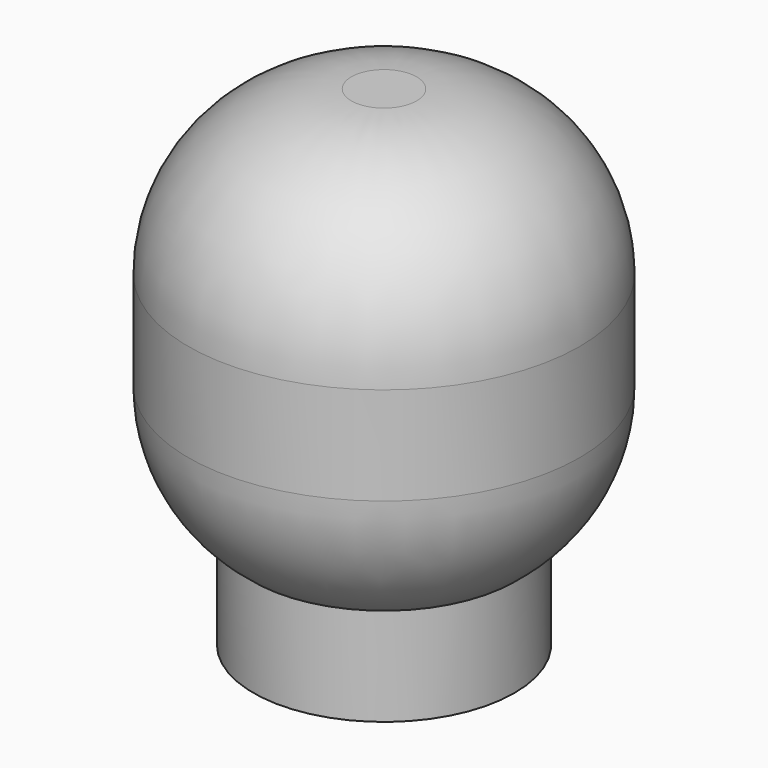
from build123d import *

# Parameters (mm, degrees)
F0_R     = 4
F1_DEPTH = 3
F2_R     = 6
F3_DEPTH = 12
F4_R     = 5
F6_R     = 2.5
F7_DEPTH = 8
F9_DEPTH = 8


# Not quite as in the source:
# - a fillet or chamfer that OpenCascade refuses, or shapes differently, is made with other operations: its cross-section is extruded or revolved along the edge and cut away or added


with BuildPart() as f1:
    # F0 (on Top) → F1 (new body)
    with BuildSketch(Plane.XY):
        Circle(F0_R)
    extrude(amount=F1_DEPTH)

    # F2 (on face) → F3 (join)
    with BuildSketch(Plane.XY.offset(3)):
        Circle(F2_R)
    extrude(amount=F3_DEPTH)

    # F4
    f4_edges = [f1.edges().sort_by_distance(p)[0] for p in [
        (-6, 0, 15),
    ]]
    fillet(f4_edges, radius=F4_R)

    # F5: fillet of radius 5 on 1 edges, made by hand

    # F5_s1 → F5_t2 (revolve, cut)
    with BuildSketch(Plane.XZ):
        with BuildLine():
            ThreePointArc((6, 7), (5.472135955, 4.7639320225), (4, 3))
            Line((4, 3), (6, 3))
            Line((6, 3), (6, 7))
        make_face()
    revolve(axis=Axis((0, 0, 3), (0, 0, 1)), mode=Mode.SUBTRACT)

    # F6 (on face) → F7 (cut)
    with BuildSketch(Plane(origin=(0, 0, 0), x_dir=(1, 0, 0), z_dir=(0, 0, -1))):
        Circle(F6_R)
    extrude(amount=-F7_DEPTH, mode=Mode.SUBTRACT)

    # F8 (on Front) → F9 (cut)
    with BuildSketch(Plane.XZ):
        with BuildLine():
            Line((-1.3463870705, 8.7240217328), (-1.3463870705, 8.3487899899))
            ThreePointArc((-1.3463870705, 8.3487899899), (-1.3369403935, 8.4423866045), (-1.3337867757, 8.5364058614))
            ThreePointArc((-1.3337867757, 8.5364058614), (-1.3369403935, 8.6304251183), (-1.3463870705, 8.7240217328))
        make_face()
        with BuildLine():
            ThreePointArc((-1.3337867757, 8.5364058614), (-1.3369403935, 8.4423866045), (-1.3463870705, 8.3487899899))
            Line((-1.3463870705, 8.3487899899), (1.4683810595, 8.3487899899))
            Line((1.4683810595, 8.3487899899), (1.4683810595, 8.5058610392))
            ThreePointArc((1.4683810595, 8.5058610392), (1.4637016301, 8.6179580539), (1.4683810595, 8.7300550686))
            Line((1.4683810595, 8.7300550686), (-1.3463870705, 8.7300550686))
            Line((-1.3463870705, 8.7300550686), (-1.3463870705, 8.7240217328))
            ThreePointArc((-1.3463870705, 8.7240217328), (-1.3369403935, 8.6304251183), (-1.3337867757, 8.5364058614))
        make_face()
        with BuildLine():
            ThreePointArc((-1.3463870705, 8.7240217328), (-4.1399498979, 8.5364058614), (-1.3463870705, 8.3487899899))
            Line((-1.3463870705, 8.3487899899), (-1.3463870705, 8.7240217328))
        make_face()
        with BuildLine():
            Line((1.4683810595, 8.7300550686), (1.4683810595, 8.5058610392))
            ThreePointArc((1.4683810595, 8.5058610392), (2.864796007, 7.2741313647), (4.1536957416, 8.6179580539))
            ThreePointArc((4.1536957416, 8.6179580539), (2.864796007, 9.9617847432), (1.4683810595, 8.7300550686))
        make_face()
        with BuildLine():
            ThreePointArc((1.4683810595, 8.7300550686), (1.4637016301, 8.6179580539), (1.4683810595, 8.5058610392))
            Line((1.4683810595, 8.5058610392), (1.4683810595, 8.7300550686))
        make_face()
    extrude(amount=-F9_DEPTH, mode=Mode.SUBTRACT)


solid = f1.part
